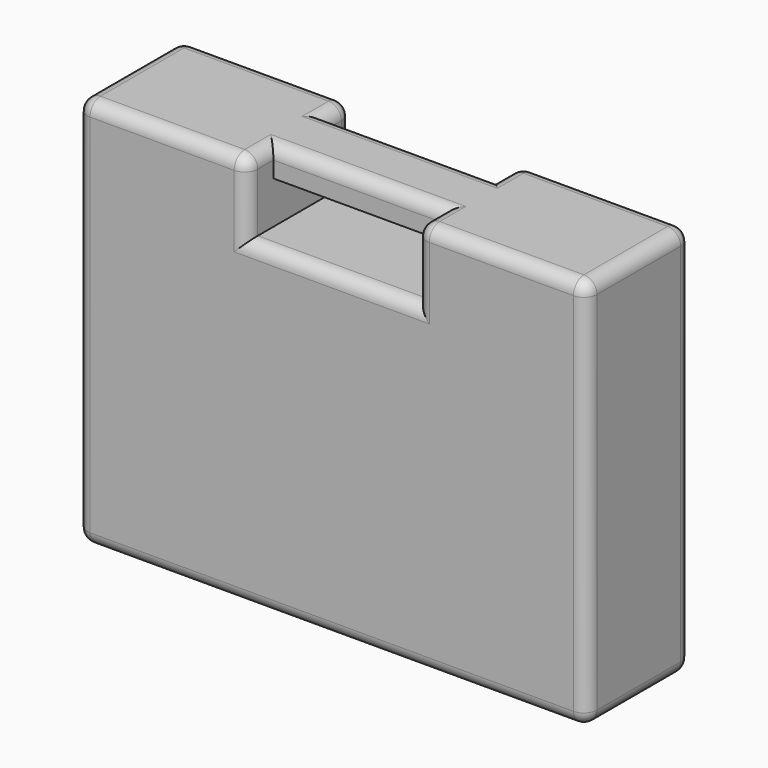
from build123d import *

# Parameters (mm, degrees)
F0_W     = 390
F0_H     = 300
F0_W_2   = 129.2868405581
F0_H_2   = 32.5715690851
F1_DEPTH = 50
F2_W     = 129.2868405581
F2_H     = 22.3345696926
F3_DEPTH = 25
F4_R     = 10


# Not quite as in the source:
# - a pattern or mirror of a feature is missing from the dataset's text; its kind, count and spacing are read off the source's solid


with BuildPart() as f1:
    # F0 (on Front) → F1 (new body, symmetric)
    with BuildSketch(Plane.XZ):
        Rectangle(F0_W, F0_H)
        with Locations((0, 111.3796457648)):
            Rectangle(F0_W_2, F0_H_2, mode=Mode.SUBTRACT)
    extrude(amount=F1_DEPTH, both=True)

    # F2 (on face) → F3 (cut)
    with BuildSketch(Plane.XZ.offset(50)):
        with Locations((0, 138.8327151537)):
            Rectangle(F2_W, F2_H)
    f3 = extrude(amount=-F3_DEPTH, mode=Mode.SUBTRACT)

    # F3_copies: F3 across plane
    add(f3.mirror(Plane.ZX), mode=Mode.SUBTRACT)

    # F4
    f4_edges = [f1.edges().sort_by_distance(p)[0] for p in [
        (0, -50, -150),
        (195, -50, 0),
        (129.82171, -50, 150),
        (64.64342, -50, 122.546931),
        (0, -50, 95.093861),
        (-64.64342, -50, 122.546931),
        (-129.82171, -50, 150),
        (-195, -50, 0),
        (-195, 0, 150),
        (-195, 50, 0),
        (-195, 0, -150),
        (195, 0, 150),
        (64.64342, -37.5, 150),
        (0, -25, 150),
        (-64.64342, -37.5, 150),
        (-129.82171, 50, 150),
        (-64.64342, 37.5, 150),
        (0, 25, 150),
        (64.64342, 37.5, 150),
        (129.82171, 50, 150),
        (0, 50, -150),
        (195, 50, 0),
        (64.64342, 50, 122.546931),
        (0, 50, 95.093861),
        (-64.64342, 50, 122.546931),
        (195, 0, -150),
    ]]
    fillet(f4_edges, radius=F4_R)


solid = f1.part
